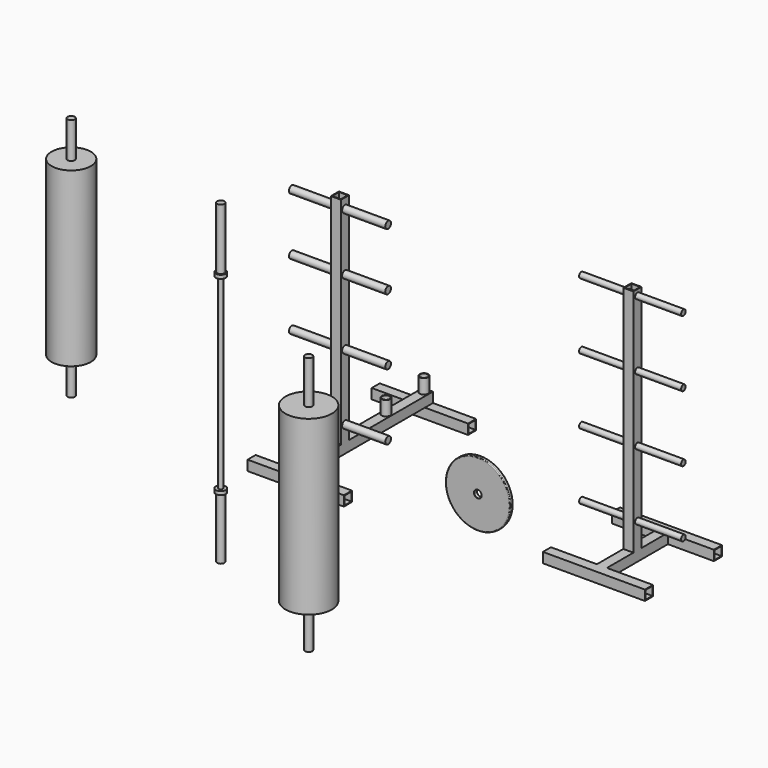
from build123d import *

# Parameters (mm, degrees)
F0_W      = 70
F0_H      = 70
F0_W_2    = 60
F0_H_2    = 60
F1_DEPTH  = 1500
F2_W      = 70
F2_H      = 1150
F3_DEPTH  = 70
F4_W      = 60
F4_H      = 60
F5_DEPTH  = 1360
F7_W      = 670
F7_H      = 70
F8_DEPTH  = 70
F9_W      = 60
F9_H      = 60
F10_DEPTH = 723
F11_R     = 30
F11_R_2   = 26
F12_DEPTH = 100
F13_R     = 25
F14_DEPTH = 300
F15_DEPTH = 370
F16_R     = 14
F17_DEPTH = 650
F18_R     = 25
F19_DEPTH = 450
F20_R     = 35
F21_DEPTH = 25
F22_DEPTH = 650
F23_R     = 25
F24_DEPTH = 450
F25_R     = 35
F26_DEPTH = 25
F27_R     = 225
F27_R_2   = 25.5
F28_DEPTH = 25
F29_R     = 5
F30_R     = 2
F31_R     = 136.5
F32_DEPTH = 1200
F33_R     = 25
F34_DEPTH = 250
F35_DEPTH = 1450
F36_W     = 70
F36_H     = 70
F37_DEPTH = 1600
F38_T     = -5
F39_W     = 70
F39_H     = 530
F40_DEPTH = 70
F41_T     = -5
F42_R     = 20
F43_DEPTH = 320
F44_DEPTH = 390
F45_R     = 161.5
F46_DEPTH = 1200
F47_R     = 25
F48_DEPTH = 300
F49_DEPTH = 1500


# Not quite as in the source:
# - a shell that OpenCascade refuses in one call is made with other operations: the cavity is built on its own and cut out


with BuildPart() as f1:
    # F0 (on Top) → F1 (new body)
    with BuildSketch(Plane.XY):
        Rectangle(F0_W, F0_H)
        Rectangle(F0_W_2, F0_H_2, mode=Mode.SUBTRACT)
    extrude(amount=F1_DEPTH)

    # F2 (on face) → F3 (join)
    with BuildSketch(Plane(origin=(0, 0, 0), x_dir=(1, 0, 0), z_dir=(0, 0, -1))):
        with Locations((0, -190)):
            Rectangle(F2_W, F2_H)
    extrude(amount=F3_DEPTH)

    # F4 (on face) → F5 (cut)
    with BuildSketch(Plane(origin=(0, 765, 0), x_dir=(-1, 0, 0), z_dir=(0, 1, 0))):
        with Locations((0, -35)):
            Rectangle(F4_W, F4_H)
    extrude(amount=-F5_DEPTH, mode=Mode.SUBTRACT)

    # F7 (on face) → F8 (join)
    with BuildSketch(Plane(origin=(0, 0, -70), x_dir=(1, 0, 0), z_dir=(0, 0, -1))):
        with Locations((0, 350)):
            Rectangle(F7_W, F7_H)
        with Locations((0, -730)):
            Rectangle(F7_W, F7_H)
    extrude(amount=F8_DEPTH)

    # F9 (on face) → F10 (cut)
    with BuildSketch(Plane(origin=(-335, 0, 0), x_dir=(0, -1, 0), z_dir=(-1, 0, 0))):
        with Locations((-730, -105)):
            Rectangle(F9_W, F9_H)
        with Locations((350, -105)):
            Rectangle(F9_W, F9_H)
    extrude(amount=-F10_DEPTH, mode=Mode.SUBTRACT)

    # F11 (on face) → F12 (join)
    with BuildSketch(Plane.XY):
        with Locations((0, -250)):
            Circle(F11_R)
        with Locations((0, -250)):
            Circle(F11_R_2, mode=Mode.SUBTRACT)
        with Locations((0, -350)):
            Circle(F11_R)
        with Locations((0, -350)):
            Circle(F11_R_2, mode=Mode.SUBTRACT)
        with Locations((0, 730)):
            Circle(F11_R)
        with Locations((0, 730)):
            Circle(F11_R_2, mode=Mode.SUBTRACT)
        with Locations((0, 400)):
            Circle(F11_R)
        with Locations((0, 400)):
            Circle(F11_R_2, mode=Mode.SUBTRACT)
    extrude(amount=F12_DEPTH)

    # F13 (on face) → F14 (join)
    with BuildSketch(Plane(origin=(-35, 0, 0), x_dir=(0, -1, 0), z_dir=(-1, 0, 0))):
        with Locations((0, 110)):
            Circle(F13_R)
        with Locations((0, 570)):
            Circle(F13_R)
        with Locations((0, 1030)):
            Circle(F13_R)
        with Locations((0, 1430)):
            Circle(F13_R)
    extrude(amount=F14_DEPTH)

    # F13 (on face) → F15 (join)
    with BuildSketch(Plane(origin=(-35, 0, 0), x_dir=(0, -1, 0), z_dir=(-1, 0, 0))):
        with Locations((0, 110)):
            Circle(F13_R)
        with Locations((0, 570)):
            Circle(F13_R)
        with Locations((0, 1030)):
            Circle(F13_R)
        with Locations((0, 1430)):
            Circle(F13_R)
    extrude(amount=-F15_DEPTH)


with BuildPart() as f17:
    # F16 (on Top) → F17 (new body)
    with BuildSketch(Plane.XY):
        with Locations((-934.9689483643, 131.9340020418)):
            Circle(F16_R)
    extrude(amount=F17_DEPTH)

    # F18 (on face) → F19 (join)
    with BuildSketch(Plane.XY.offset(650)):
        with Locations((-934.9689483643, 131.9340020418)):
            Circle(F18_R)
    extrude(amount=F19_DEPTH)

    # F20 (on face) → F21 (join)
    with BuildSketch(Plane(origin=(0, 0, 650), x_dir=(1, 0, 0), z_dir=(0, 0, -1))):
        with Locations((-934.9689483643, -131.9340020418)):
            Circle(F20_R)
    extrude(amount=-F21_DEPTH)

    # F16 (on Top) → F22 (join)
    with BuildSketch(Plane.XY):
        with Locations((-934.9689483643, 131.9340020418)):
            Circle(F16_R)
    extrude(amount=-F22_DEPTH)

    # F23 (on face) → F24 (join)
    with BuildSketch(Plane(origin=(0, 0, -650), x_dir=(1, 0, 0), z_dir=(0, 0, -1))):
        with Locations((-934.9689483643, -131.9340020418)):
            Circle(F23_R)
    extrude(amount=F24_DEPTH)

    # F25 (on face) → F26 (join)
    with BuildSketch(Plane.XY.offset(-650)):
        with Locations((-934.9689483643, 131.9340020418)):
            Circle(F25_R)
    extrude(amount=-F26_DEPTH)


with BuildPart() as f28:
    # F27 (on Front) → F28 (new body)
    with BuildSketch(Plane.XZ):
        with Locations((979.3181844601, 0)):
            Circle(F27_R)
        with Locations((979.3181844601, 0)):
            Circle(F27_R_2, mode=Mode.SUBTRACT)
    extrude(amount=F28_DEPTH)

    # F29
    f29_edges = [f28.edges().sort_by_distance(p)[0] for p in [
        (754.318184, 0, 0),
        (754.318184, -25, 0),
    ]]
    fillet(f29_edges, radius=F29_R)

    # F30
    f30_edges = [f28.edges().sort_by_distance(p)[0] for p in [
        (953.818184, 0, 0),
        (953.818184, -25, 0),
    ]]
    fillet(f30_edges, radius=F30_R)


with BuildPart() as f32:
    # F31 (on Top) → F32 (new body)
    with BuildSketch(Plane.XY):
        with Locations((-1770.6463336945, -124.7432902455)):
            Circle(F31_R)
    extrude(amount=F32_DEPTH)

    # F33 (on face) → F34 (join)
    with BuildSketch(Plane.XY.offset(1200)):
        with Locations((-1770.6463336945, -124.7432902455)):
            Circle(F33_R)
    extrude(amount=F34_DEPTH)

    # F33 (on face) → F35 (join)
    with BuildSketch(Plane.XY.offset(1200)):
        with Locations((-1770.6463336945, -124.7432902455)):
            Circle(F33_R)
    extrude(amount=-F35_DEPTH)


with BuildPart() as f37:
    # F36 (on Top) → F37 (new body)
    with BuildSketch(Plane.XY):
        with Locations((2035, 0)):
            Rectangle(F36_W, F36_H)
    extrude(amount=F37_DEPTH)

    # F38
    f38_openings = [f37.faces().sort_by_distance(p)[0] for p in [
        (2035, 0, 1600),
        (2035, 0, 0),
    ]]
    offset(amount=F38_T, openings=f38_openings)

    # F39 (on face) → F40 (join)
    with BuildSketch(Plane(origin=(0, 0, 0), x_dir=(1, 0, 0), z_dir=(0, 0, -1))):
        Polygon((1680, 265), (2000, 265), (2070, 265), (2390, 265), (2390, 335), (1680, 335), align=None)
        with Locations((2035, 0)):
            Rectangle(F39_W, F39_H)
        Polygon((2070, -265), (2000, -265), (1680, -265), (1680, -335), (2390, -335), (2390, -265), align=None)
    extrude(amount=F40_DEPTH)

    # F41: a shell. OpenCascade refuses it in one call, so the cavity is built on its own and cut out:
    # the body offset inwards by the wall thickness, plus a prism from it out through each open face.
    f41_core = offset(f37.part, amount=F41_T, kind=Kind.INTERSECTION, mode=Mode.PRIVATE)
    f41_exits = [f41_core.faces().sort_by_distance(p)[0] for p in [
        (2385, -300, -35),
        (2385, 300, -35),
        (1685, 300, -35),
        (1685, -300, -35),
    ]]
    add(f41_core, mode=Mode.SUBTRACT)
    extrude(f41_exits, amount=-F41_T, mode=Mode.SUBTRACT)

    # F42 (on face) → F43 (join)
    with BuildSketch(Plane.YZ.offset(2070)):
        with Locations((0, 180)):
            Circle(F42_R)
        with Locations((0, 640)):
            Circle(F42_R)
        with Locations((0, 1100)):
            Circle(F42_R)
        with Locations((0, 1560)):
            Circle(F42_R)
    extrude(amount=F43_DEPTH)

    # F42 (on face) → F44 (join)
    with BuildSketch(Plane.YZ.offset(2070)):
        with Locations((0, 180)):
            Circle(F42_R)
        with Locations((0, 640)):
            Circle(F42_R)
        with Locations((0, 1100)):
            Circle(F42_R)
        with Locations((0, 1560)):
            Circle(F42_R)
    extrude(amount=-F44_DEPTH)


with BuildPart() as f46:
    # F45 (on Top) → F46 (new body)
    with BuildSketch(Plane.XY):
        with Locations((1047.1220016479, -1581.1581611633)):
            Circle(F45_R)
    extrude(amount=F46_DEPTH)

    # F47 (on face) → F48 (join)
    with BuildSketch(Plane.XY.offset(1200)):
        with Locations((1047.1220016479, -1581.1581611633)):
            Circle(F47_R)
    extrude(amount=F48_DEPTH)

    # F47 (on face) → F49 (join)
    with BuildSketch(Plane.XY.offset(1200)):
        with Locations((1047.1220016479, -1581.1581611633)):
            Circle(F47_R)
    extrude(amount=-F49_DEPTH)


solid = Compound([f1.part, f17.part, f28.part, f32.part, f37.part, f46.part])
